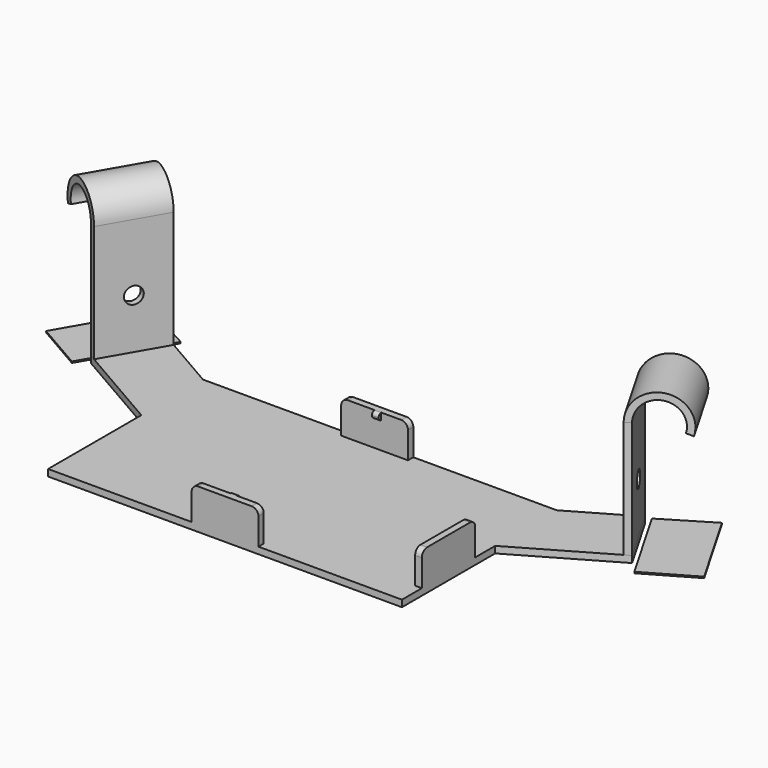
from build123d import *

# Parameters (mm, degrees)
F1_DEPTH  = 2
F3_DEPTH  = 35
F5_DEPTH  = 20
F6_W      = 6.5
F6_H      = 2
F7_DEPTH  = 20
F9_DEPTH  = 20
F10_W     = 6.5
F10_H     = 2
F11_DEPTH = 20
F12_R     = 2.5
F13_DEPTH = 2
F14_R     = 2.5
F15_DEPTH = 2
F16_W     = 20
F16_H     = 2
F16_W_2   = 2
F16_H_2   = 20
F17_DEPTH = 10
F18_R     = 2
F19_W     = 2
F19_H     = 2
F20_DEPTH = 1
F21_R     = 0.99999
F22_W     = 2
F22_H     = 2
F23_DEPTH = 1
F24_R     = 0.99999
F26_DEPTH = 0.4


# Not quite as in the source:
# - a fillet or chamfer is up to 0.001 mm smaller than in the source, because OpenCascade refuses the exact size


with BuildPart() as f1:
    # F0 (on Top) → F1 (new body)
    with BuildSketch(Plane.XY):
        Polygon((-67.9032802582, 30.168056488), (38.0967197418, 30.168056488), (38.0967197418, 65.0740457205), (38.0967197418, 88.168056488), (-67.9032802582, 88.168056488), (-67.9032802582, 65.0740457205), align=None)
        Polygon((-101.5896410854, 84.5228752121), (-67.9032802582, 65.0740457205), (-67.9032802582, 88.168056488), (-91.5896410854, 101.8433832877), align=None)
        Polygon((38.0967197418, 88.168056488), (38.0967197418, 65.0740457205), (71.783080569, 84.5228752121), (61.783080569, 101.8433832877), align=None)
    extrude(amount=F1_DEPTH)

    # F2 (on face) → F3 (join)
    with BuildSketch(Plane.XY.offset(2)):
        Polygon((-84.2284251532, 97.5933832877), (-85.9604759608, 98.5933832877), (-95.9604759608, 81.2728752121), (-94.2284251532, 80.2728752121), align=None)
        Polygon((56.1539154444, 98.5933832877), (54.4218646369, 97.5933832877), (64.4218646369, 80.2728752121), (66.1539154444, 81.2728752121), align=None)
    extrude(amount=F3_DEPTH)

    # F4 (on face) → F5 (join)
    with BuildSketch(Plane(origin=(-18.653708425, 32.3091707417, 0), x_dir=(0.8660254038, 0.5, 0), z_dir=(0.5, -0.8660254038, 0))):
        with BuildLine():
            ThreePointArc((97.9274089407, 37), (105.3169745916, 43.4388409635), (110.6839236954, 35.2376086915))
            Line((110.6839236954, 35.2376086915), (112.5673020138, 34.5521150438))
            ThreePointArc((112.5673020138, 34.5521150438), (105.664524311, 45.4094913973), (95.9274089407, 37))
            Line((95.9274089407, 37), (97.9274089407, 37))
        make_face()
    extrude(amount=-F5_DEPTH)

    # F6 (on face) → F7 (cut)
    with BuildSketch(Plane(origin=(-18.653708425, 32.3091707417, 0), x_dir=(0.8660254038, 0.5, 0), z_dir=(0.5, -0.8660254038, 0))):
        with Locations((101.1774089407, 1)):
            Rectangle(F6_W, F6_H)
    extrude(amount=-F7_DEPTH, mode=Mode.SUBTRACT)

    # F8 (on face) → F9 (join)
    with BuildSketch(Plane(origin=(11.2020682959, 19.4025514384, 0), x_dir=(0.8660254038, -0.5, 0), z_dir=(-0.5, -0.8660254038, 0))):
        Polygon((-121.7406475473, 2), (-121.7406475473, 37), (-123.7406475473, 37), (-123.7406475473, 2), (-130.2406475473, 2), (-130.2406475473, 0), (-91.3429885641, 0), (-91.3429885641, 2), align=None)
        with BuildLine():
            Line((-123.7406475473, 37), (-121.7406475473, 37))
            ThreePointArc((-121.7406475473, 37), (-131.2541063524, 45.439366164), (-138.4989772533, 34.9875411887))
            Line((-138.4989772533, 34.9875411887), (-136.6045913116, 35.6770412837))
            ThreePointArc((-136.6045913116, 35.6770412837), (-130.9056157917, 43.4658964757), (-123.7406475473, 37))
        make_face()
    extrude(amount=-F9_DEPTH)

    # F10 (on face) → F11 (cut)
    with BuildSketch(Plane(origin=(11.2020682959, 19.4025514384, 0), x_dir=(0.8660254038, -0.5, 0), z_dir=(-0.5, -0.8660254038, 0))):
        with Locations((-126.9906475473, 1)):
            Rectangle(F10_W, F10_H)
    extrude(amount=-F11_DEPTH, mode=Mode.SUBTRACT)

    # F12 (on face) → F13 (cut)
    with BuildSketch(Plane(origin=(-105.4304934491, 60.8703237737, 0), x_dir=(0.5, 0.8660254038, 0), z_dir=(0.8660254038, -0.5, 0))):
        with Locations((32.4041365919, 17)):
            Circle(F12_R)
    extrude(amount=-F13_DEPTH, mode=Mode.SUBTRACT)

    # F14 (on face) → F15 (cut)
    with BuildSketch(Plane(origin=(83.0755730619, 47.9637044704, 0), x_dir=(0.5, -0.8660254038, 0), z_dir=(-0.8660254038, -0.5, 0))):
        with Locations((-47.30741685, 17)):
            Circle(F14_R)
    extrude(amount=-F15_DEPTH, mode=Mode.SUBTRACT)

    # F16 (on face) → F17 (join)
    with BuildSketch(Plane.XY.offset(2)):
        with Locations((-14.9032802582, 87.168056488)):
            Rectangle(F16_W, F16_H)
        with Locations((-14.9032802582, 31.168056488)):
            Rectangle(F16_W, F16_H)
        with Locations((37.0967197418, 47.6210511042)):
            Rectangle(F16_W_2, F16_H_2)
    extrude(amount=F17_DEPTH)

    # F18
    f18_edges = [f1.edges().sort_by_distance(p)[0] for p in [
        (-24.90328, 87.168056, 12),
        (-4.90328, 87.168056, 12),
        (-24.90328, 31.168056, 12),
        (-4.90328, 31.168056, 12),
        (37.09672, 37.621051, 12),
        (37.09672, 57.621051, 12),
    ]]
    fillet(f18_edges, radius=F18_R)

    # F19 (on face) → F20 (join)
    with BuildSketch(Plane.XZ.offset(-86.168056488)):
        with Locations((-13.9032802582, 11)):
            Rectangle(F19_W, F19_H)
    extrude(amount=F20_DEPTH)

    # F21 (radius 1 in the source; OpenCascade refuses exactly that, so slightly less here)
    f21_edges = [f1.edges().sort_by_distance(p)[0] for p in [
        (-13.90328, 85.168056, 10),
        (-13.90328, 85.168056, 12),
    ]]
    fillet(f21_edges, radius=F21_R)

    # F22 (on face) → F23 (join)
    with BuildSketch(Plane(origin=(0, 32.168056488, 0), x_dir=(-1, 0, 0), z_dir=(0, 1, 0))):
        with Locations((13.9032802582, 11)):
            Rectangle(F22_W, F22_H)
    extrude(amount=F23_DEPTH)

    # F24 (radius 1 in the source; OpenCascade refuses exactly that, so slightly less here)
    f24_edges = [f1.edges().sort_by_distance(p)[0] for p in [
        (-13.90328, 33.168056, 10),
        (-13.90328, 33.168056, 12),
    ]]
    fillet(f24_edges, radius=F24_R)


with BuildPart() as f26:
    # F25 (on face) → F26 (new body)
    with BuildSketch(Plane(origin=(0, 0, 0), x_dir=(1, 0, 0), z_dir=(0, 0, -1))):
        Polygon((69.792699928, -77.5712246278), (56.1539154444, -101.1942923069), (70.3034838034, -109.7310148019), (84.1013854701, -85.8323480773), align=None)
    extrude(amount=-F26_DEPTH)


with BuildPart() as f26b:
    # F25 (on face) → F26, piece 2 (new body)
    with BuildSketch(Plane(origin=(0, 0, 0), x_dir=(1, 0, 0), z_dir=(0, 0, -1))):
        Polygon((-100.3888883417, -110.1487811715), (-85.8259052038, -102.2308915854), (-99.4944213659, -78.5563271285), (-113.8452054823, -86.8417562012), align=None)
    extrude(amount=-F26_DEPTH)


solid = Compound([f1.part, f26.part, f26b.part])
